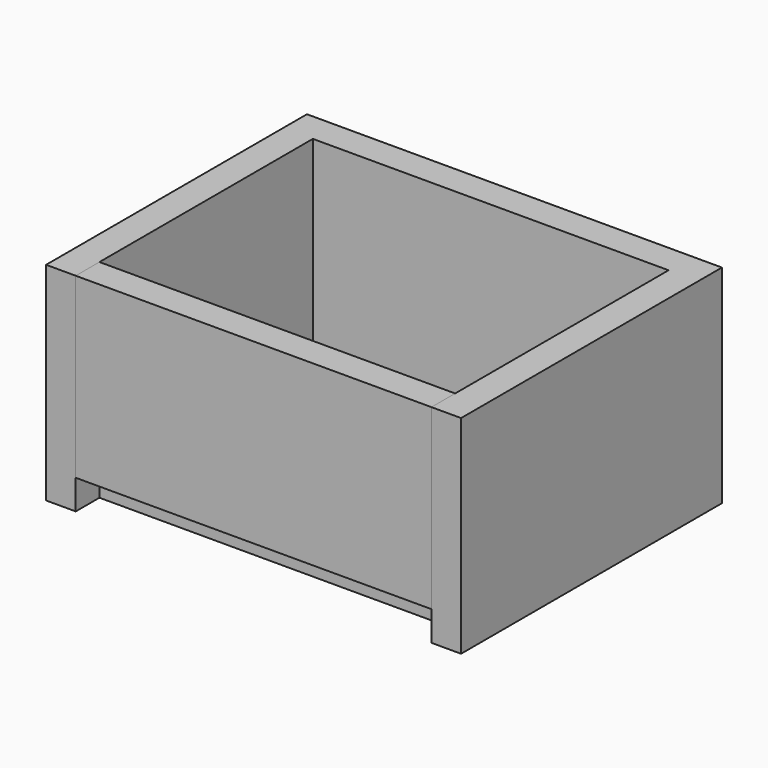
from build123d import *

# Parameters (mm, degrees)
F0_W          = 304.8
F0_H          = 228.6
F1_DEPTH      = 25.4
F2_DEPTH      = 152.4
F2_DEPTH_BACK = 25.4
F0_H_2        = 25.4
F3_DEPTH      = 152.4
F4_R          = 6.35
F4_R_2        = 3.175
F5_DEPTH      = 304.8
F6_DEPTH      = 304.8
F7_DEPTH      = 304.8
F8_W          = 50.8
F8_H          = 31.75
F10_DEPTH     = 3.175
F9_W          = 50.8
F9_H          = 31.75
F9_W_2        = 50.8000000005
F11_DEPTH     = 3.175


with BuildPart() as f1:
    # F0 (on Top) → F1 (new body)
    with BuildSketch(Plane.XY):
        with Locations((152.4, 114.3)):
            Rectangle(F0_W, F0_H)
    extrude(amount=-F1_DEPTH)

    # F0 (on Top) → F2 (join, two sides)
    with BuildSketch(Plane.XY) as f2_sk:
        Polygon((0, -25.4), (0, 0), (0, 228.6), (304.8, 228.6), (304.8, 0), (304.8, -25.4), (330.2, -25.4), (330.2, 254), (-25.4, 254), (-25.4, -25.4), align=None)
    extrude(amount=F2_DEPTH)
    extrude(f2_sk.sketch, amount=-F2_DEPTH_BACK)


with BuildPart() as f3:
    # F0 (on Top) → F3 (new body)
    with BuildSketch(Plane.XY):
        with Locations((152.4, -12.7)):
            Rectangle(F0_W, F0_H_2)
    extrude(amount=F3_DEPTH)


with BuildPart() as f5_tool:
    # F4 (on Right) → F5 (new body, through all)
    with BuildSketch(Plane.YZ):
        Circle(F4_R)
        Circle(F4_R_2, mode=Mode.SUBTRACT)
        Circle(F4_R_2)
    extrude(amount=F5_DEPTH)


with BuildPart() as f1_1:
    add(f1.part)

    # F5: cut by f5_tool
    add(f5_tool.part, mode=Mode.SUBTRACT)

    # F4 (on Right) → F6 (join, through all)
    with BuildSketch(Plane.YZ):
        Circle(F4_R_2)
    extrude(amount=F6_DEPTH)


with BuildPart() as f3_1:
    add(f3.part)

    # F5: cut by f5_tool
    add(f5_tool.part, mode=Mode.SUBTRACT)


with BuildPart() as f7:
    # F4 (on Right) → F7 (new body, through all)
    with BuildSketch(Plane.YZ):
        Circle(F4_R)
        Circle(F4_R_2, mode=Mode.SUBTRACT)
    extrude(amount=F7_DEPTH)

    # F8 (on face) → F10 (join)
    with BuildSketch(Plane(origin=(0, 0, 0), x_dir=(-1, 0, 0), z_dir=(0, 1, 0))):
        with Locations((-279.4, 15.875)):
            Rectangle(F8_W, F8_H)
        with Locations((-177.8, 15.875)):
            Rectangle(F8_W, F8_H)
        with Locations((-76.2, 15.875)):
            Rectangle(F8_W, F8_H)
    extrude(amount=F10_DEPTH)

    # F9 (on face) → F11 (join)
    with BuildSketch(Plane.XY):
        with Locations((25.4, 15.875)):
            Rectangle(F9_W, F9_H)
        with Locations((127.0000000002, 15.875)):
            Rectangle(F9_W_2, F9_H)
        with Locations((228.6, 15.875)):
            Rectangle(F9_W, F9_H)
    extrude(amount=F11_DEPTH)


solid = Compound([f1_1.part, f3_1.part, f7.part])
